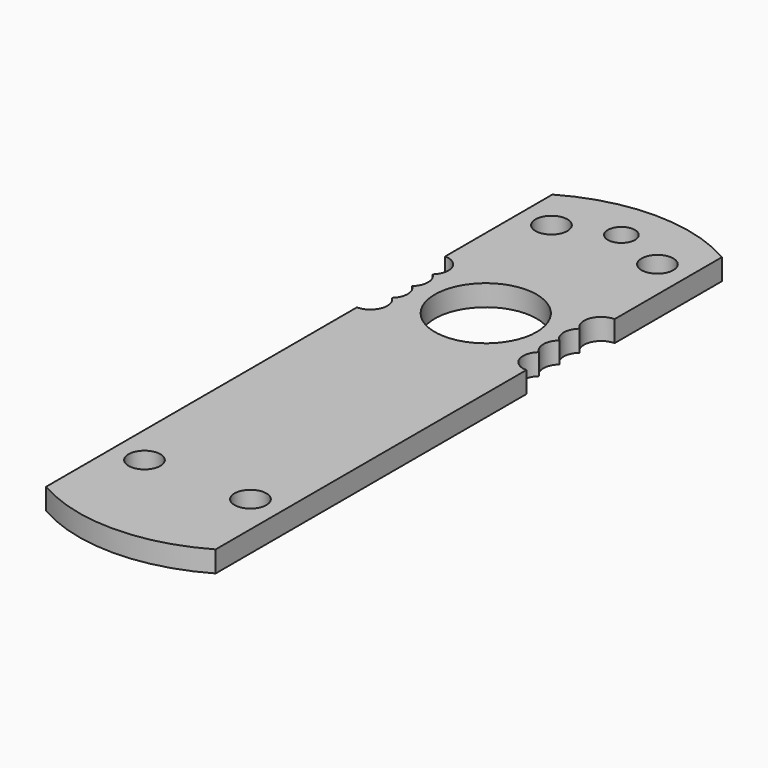
from build123d import *

# Parameters (mm, degrees)
F1_DEPTH = 3.175
F2_R     = 2.38125
F3_DEPTH = 3.175
F4_R     = 7.62
F4_R_2   = 2.032
F5_DEPTH = 25.4


# Not quite as in the source:
# - a feature names something its author has since deleted; it is built from what else it names


with BuildPart() as f1:
    # F0 (on Top) → F1 (new body)
    with BuildSketch(Plane.XY):
        with BuildLine():
            Line((12.7, 0), (12.7, 47.3970452561))
            ThreePointArc((12.7, 47.3970452561), (0, 50.8), (-12.7, 47.3970452561))
            Line((-12.7, 47.3970452561), (-12.7, 0))
            Line((-12.7, 0), (0, 0))
            Line((0, 0), (12.7, 0))
        make_face()
        with BuildLine():
            Line((12.7, -47.3970452561), (12.7, 0))
            Line((12.7, 0), (0, 0))
            Line((0, 0), (-12.7, 0))
            Line((-12.7, 0), (-12.7, -47.3970452561))
            ThreePointArc((-12.7, -47.3970452561), (0, -50.8), (12.7, -47.3970452561))
        make_face()
    extrude(amount=F1_DEPTH)

    # F2 (on face) → F3 (cut, through all)
    with BuildSketch(Plane.XY.offset(3.175)):
        with Locations((-7.9375, 41.275)):
            Circle(F2_R)
        with Locations((7.9375, 41.275)):
            Circle(F2_R)
        with Locations((-7.9375, -34.925)):
            Circle(F2_R)
        with Locations((7.9375, -34.925)):
            Circle(F2_R)
    extrude(amount=-F3_DEPTH, mode=Mode.SUBTRACT)

    # F4 (on face) → F5 (cut)
    with BuildSketch(Plane.XY.offset(3.175)):
        with Locations((0, 19.05)):
            Circle(F4_R)
        with BuildLine():
            ThreePointArc((-11.0199479175, 19.05), (-10.16, 20.955), (-11.0199479175, 22.86))
            ThreePointArc((-11.0199479175, 22.86), (-10.3240475594, 25.6630256121), (-12.7, 27.305))
            Line((-12.7, 27.305), (-12.7, 23.495))
            Line((-12.7, 23.495), (-12.7, 22.225))
            Line((-12.7, 22.225), (-12.7, 19.685))
            Line((-12.7, 19.685), (-12.7, 18.415))
            Line((-12.7, 18.415), (-12.7, 15.875))
            Line((-12.7, 15.875), (-12.7, 14.605))
            Line((-12.7, 14.605), (-12.7, 10.795))
            ThreePointArc((-12.7, 10.795), (-10.3240475594, 12.4369743879), (-11.0199479175, 15.24))
            ThreePointArc((-11.0199479175, 15.24), (-10.16, 17.145), (-11.0199479175, 19.05))
        make_face()
        with BuildLine():
            Line((12.7, 10.795), (12.7, 27.305))
            ThreePointArc((12.7, 27.305), (10.3240475594, 25.6630256121), (11.0199479175, 22.86))
            ThreePointArc((11.0199479175, 22.86), (10.16, 20.955), (11.0199479175, 19.05))
            ThreePointArc((11.0199479175, 19.05), (10.16, 17.145), (11.0199479175, 15.24))
            ThreePointArc((11.0199479175, 15.24), (10.3240475594, 12.4369743879), (12.7, 10.795))
        make_face()
        with Locations((0, 44.45)):
            Circle(F4_R_2)
    extrude(amount=-F5_DEPTH, mode=Mode.SUBTRACT)


solid = f1.part
